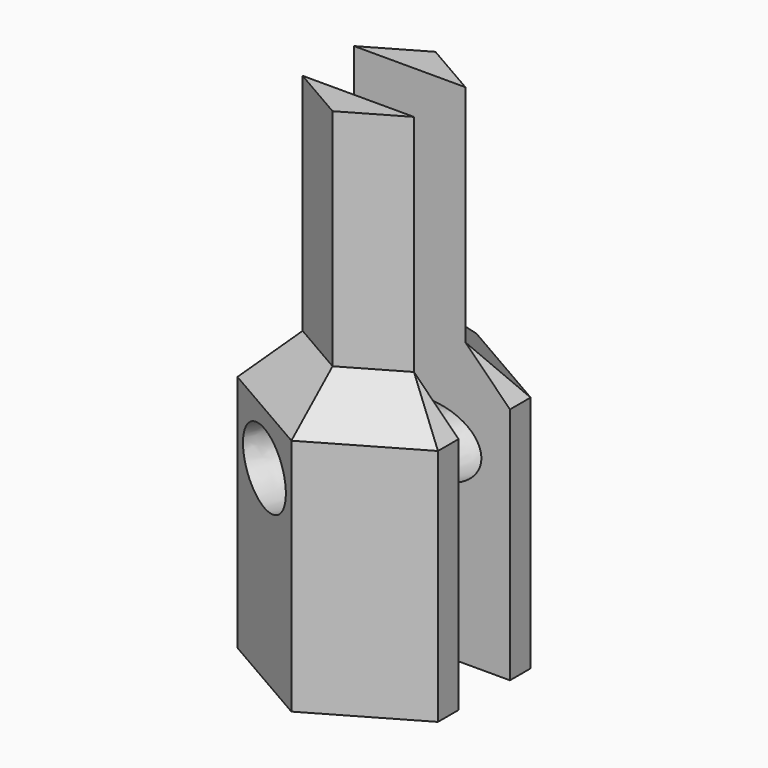
from build123d import *

# Parameters (mm, degrees)
F1_DEPTH  = 127
F2_SIZE   = 20
F3_DEPTH  = 100.7419452071
F4_W      = 73.9247704289
F4_H      = 28.8404997019
F5_DEPTH  = 227.7429452071
F10_DEPTH = 112.4425134991


# Not quite as in the source:
# - the program builds the solid bodies; features that only make, move or delete a surface that nothing else refers to are left out


with BuildPart() as f1:
    # F0 (on Top) → F1 (new body)
    with BuildSketch(Plane.XY):
        Polygon((-44.9766053996, -25.9672552347), (0, -51.9345104694), (44.9766053996, -25.9672552347), (44.9766053996, 25.9672552347), (0, 51.9345104694), (-44.9766053996, 25.9672552347), align=None)
    extrude(amount=F1_DEPTH)

    # F2
    f2_edges = [f1.edges().sort_by_distance(p)[0] for p in [
        (-44.976605, 0, 127),
        (-22.488303, 38.950883, 127),
        (22.488303, 38.950883, 127),
        (44.976605, 0, 127),
        (22.488303, -38.950883, 127),
        (-22.488303, -38.950883, 127),
    ]]
    chamfer(f2_edges, length=F2_SIZE)

    # F3 (add): a face of the model
    f3_faces = [f1.faces().sort_by_distance(p)[0] for p in [
        (0, 0, 127),
    ]]
    extrude(f3_faces, amount=F3_DEPTH)

    # F4 (on face) → F5 (cut, through all)
    with BuildSketch(Plane.XY.offset(227.7419452071)):
        with Locations((11.9857798148, 0)):
            Rectangle(F4_W, F4_H)
    extrude(amount=-F5_DEPTH, mode=Mode.SUBTRACT)

    # F8 (on face) → F10 (cut, through all)
    with BuildSketch(Plane(origin=(-22.4883026998, -38.9508828521, 0), x_dir=(0.8660254038, -0.5, 0), z_dir=(-0.5, -0.8660254038, 0))):
        with BuildLine():
            add(Edge.make_bspline(
                [(0, 67.8614079952), (35.7205863144, 67.8614079952), (17.8602931572, 91.3859009743), (0, 114.9103939533), (-17.8602931572, 91.3859009743), (-35.7205863144, 67.8614079952), (0, 67.8614079952)],
                knots=[4.7123889804, 4.7123889804, 4.7123889804, 6.8067840828, 6.8067840828, 8.9011791852, 8.9011791852, 10.9955742876, 10.9955742876, 10.9955742876], degree=2, weights=[1, 0.5, 1, 0.5, 1, 0.5, 1]))
        make_face()
    extrude(amount=-F10_DEPTH, mode=Mode.SUBTRACT)


solid = f1.part
